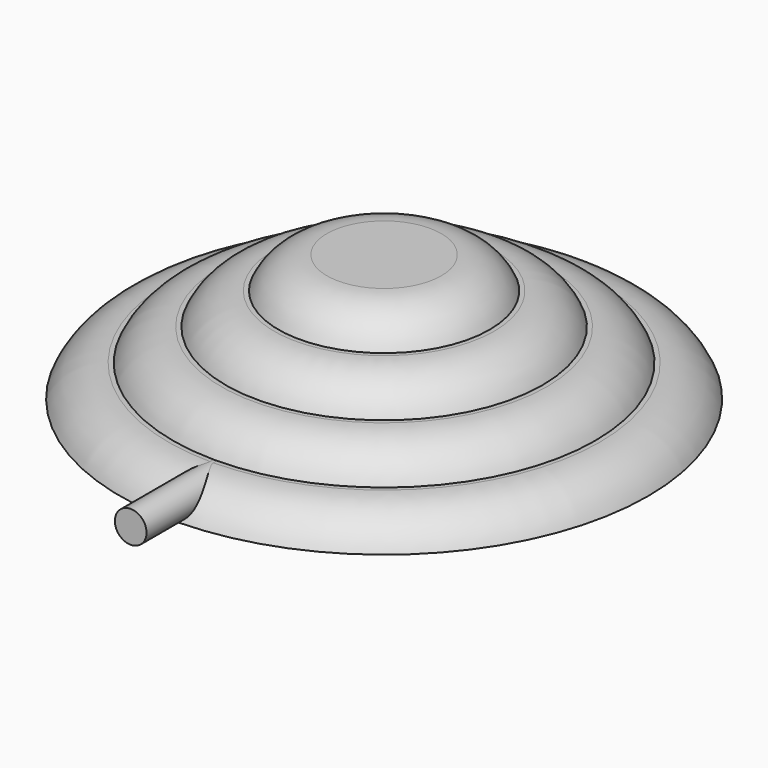
from build123d import *

# Parameters (mm, degrees)
F0_R      = 25
F2_DEPTH  = 3
F1_R      = 20
F3_DEPTH  = 6
F4_R      = 15
F5_DEPTH  = 9
F6_R      = 10
F7_DEPTH  = 12
F12_R     = 1.5
F13_DEPTH = 30


# Not quite as in the source:
# - a fillet or chamfer that OpenCascade refuses, or shapes differently, is made with other operations: its cross-section is extruded or revolved along the edge and cut away or added


with BuildPart() as f2:
    # F0 (on Top) → F2 (new body)
    with BuildSketch(Plane.XY):
        Circle(F0_R)
    extrude(amount=F2_DEPTH)

    # F1 (on Top) → F3 (join)
    with BuildSketch(Plane.XY):
        Circle(F1_R)
    extrude(amount=F3_DEPTH)

    # F4 (on Top) → F5 (join)
    with BuildSketch(Plane.XY):
        Circle(F4_R)
    extrude(amount=F5_DEPTH)

    # F6 (on Top) → F7 (join)
    with BuildSketch(Plane.XY):
        Circle(F6_R)
    extrude(amount=F7_DEPTH)

    # F8: fillet of radius 5 on 1 edges, made by hand

    # F8_s1 → F8_t2 (revolve, cut)
    with BuildSketch(Plane.XZ):
        with BuildLine():
            ThreePointArc((10, 9), (8.1560370926, 11.1833001327), (5.417424305, 12))
            Line((5.417424305, 12), (10, 12))
            Line((10, 12), (10, 9))
        make_face()
    revolve(axis=Axis((0, 0, 12), (0, 0, 1)), mode=Mode.SUBTRACT)

    # F9: fillet of radius 5 on 1 edges, made by hand

    # F9_s1 → F9_t2 (revolve, cut)
    with BuildSketch(Plane.XZ):
        with BuildLine():
            ThreePointArc((15, 6), (13.1560370926, 8.1833001327), (10.417424305, 9))
            Line((10.417424305, 9), (15, 9))
            Line((15, 9), (15, 6))
        make_face()
    revolve(axis=Axis((0, 0, 9), (0, 0, 1)), mode=Mode.SUBTRACT)

    # F10: fillet of radius 5 on 1 edges, made by hand

    # F10_s1 → F10_t2 (revolve, cut)
    with BuildSketch(Plane.XZ):
        with BuildLine():
            ThreePointArc((20, 3), (18.1560370926, 5.1833001327), (15.417424305, 6))
            Line((15.417424305, 6), (20, 6))
            Line((20, 6), (20, 3))
        make_face()
    revolve(axis=Axis((0, 0, 6), (0, 0, 1)), mode=Mode.SUBTRACT)

    # F11: fillet of radius 5 on 1 edges, made by hand

    # F11_s1 → F11_t2 (revolve, cut)
    with BuildSketch(Plane.XZ):
        with BuildLine():
            ThreePointArc((25, 0), (23.1560370926, 2.1833001327), (20.417424305, 3))
            Line((20.417424305, 3), (25, 3))
            Line((25, 3), (25, 0))
        make_face()
    revolve(axis=Axis((0, 0, 3), (0, 0, 1)), mode=Mode.SUBTRACT)

    # F12 (on Front) → F13 (join)
    with BuildSketch(Plane.XZ):
        with Locations((0, 1.508576342)):
            Circle(F12_R)
    extrude(amount=F13_DEPTH)


solid = f2.part
